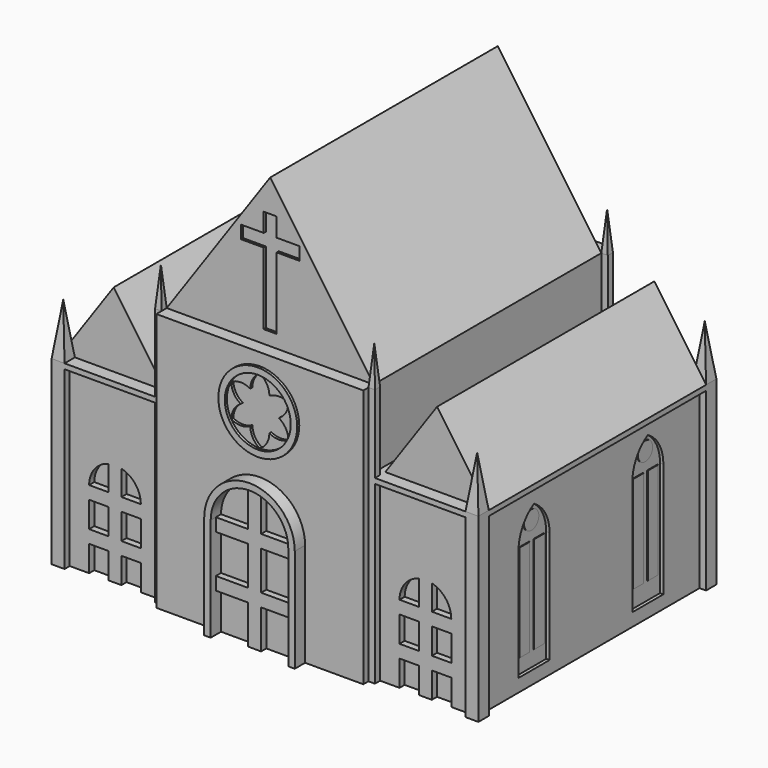
from build123d import *

# Parameters (mm, degrees)
F0_W      = 3.175
F0_H      = 3.175
F1_DEPTH  = 127
F2_DEPTH  = 88.9
F3_W      = 50.8
F3_H      = 146.05
F4_DEPTH  = 2.54
F5_W      = 3.175
F5_H      = 133.35
F5_W_2    = 44.45
F5_H_2    = 3.175
F6_DEPTH  = 2.54
F8_DEPTH  = 139.7
F10_DEPTH = 139.7
F12_DEPTH = 146.05
F13_DEPTH = 6.35
F14_DEPTH = 6.35
F15_DEPTH = 6.35
F17_DEPTH = 3.175
F19_DEPTH = 3.175
F21_DEPTH = 127
F23_DEPTH = 3.175
F25_DEPTH = 3.175
F27_DEPTH = 127
F29_DEPTH = 6.35
F31_DEPTH = 25.4
F33_DEPTH = 6.35
F35_DEPTH = 14.732
F37_DEPTH = 6.35
F39_DEPTH = 25.4
F41_DEPTH = 6.35
F43_DEPTH = 6.35
F45_DEPTH = 6.35
F47_DEPTH = 3.175
F48_W     = 6.35
F48_H     = 6.35
F48_H_2   = 9.202644515
F48_W_2   = 11.1125
F48_H_3   = 35.247355485
F49_DEPTH = 1.27
F50_R     = 19.3618203149
F51_DEPTH = 1.27
F53_DEPTH = 1.27
F54_W     = 9.525
F54_H     = 12.7
F55_DEPTH = 3.175
F56_W     = 9.525
F56_H     = 12.7
F57_DEPTH = 3.175
F58_W     = 6.35
F58_H     = 47.625
F58_R     = 4.5339
F60_DEPTH = 1.651
F59_W     = 6.35
F59_H     = 47.625
F59_R     = 4.5339
F61_DEPTH = 1.27
F62_DEPTH = 1.651
F63_DEPTH = 1.27
F64_W     = 6.35
F64_H     = 47.625
F64_R     = 4.5339
F66_DEPTH = 1.27
F67_DEPTH = 1.4224
F65_R     = 4.5339
F65_W     = 6.35
F65_H     = 47.625
F68_DEPTH = 1.27
F69_DEPTH = 1.4224
F71_DEPTH = 6.35
F70_W     = 19.05
F70_H     = 25.4
F72_DEPTH = 3.175


# Not quite as in the source:
# - a pattern or mirror of a feature is missing from the dataset's text; its kind, count and spacing are read off the source's solid


with BuildPart() as f1:
    # F0 (on Top) → F1 (new body)
    with BuildSketch(Plane.XY):
        Polygon((50.8, 76.2), (-50.8, 76.2), (-50.8, 73.025), (-50.8, 69.85), (-50.8, -69.85), (-50.8, -73.025), (-50.8, -76.2), (50.8, -76.2), (50.8, -73.025), (50.8, -69.85), (50.8, 69.85), (50.8, 73.025), align=None)
        with Locations((-52.3875, 71.4375)):
            Rectangle(F0_W, F0_H)
        with Locations((52.3875, 71.4375)):
            Rectangle(F0_W, F0_H)
        with Locations((-52.3875, -71.4375)):
            Rectangle(F0_W, F0_H)
        with Locations((52.3875, -71.4375)):
            Rectangle(F0_W, F0_H)
    extrude(amount=F1_DEPTH)

    # F0 (on Top) → F2 (join)
    with BuildSketch(Plane.XY):
        with Locations((-52.3875, -71.4375)):
            Rectangle(F0_W, F0_H)
        Polygon((50.8, 76.2), (-50.8, 76.2), (-50.8, 73.025), (-50.8, 69.85), (-50.8, -69.85), (-50.8, -73.025), (-50.8, -76.2), (50.8, -76.2), (50.8, -73.025), (50.8, -69.85), (50.8, 69.85), (50.8, 73.025), align=None)
        with Locations((-52.3875, 71.4375)):
            Rectangle(F0_W, F0_H)
        Polygon((53.975, 69.85), (50.8, 69.85), (50.8, -69.85), (53.975, -69.85), (98.425, -69.85), (98.425, -73.025), (104.775, -73.025), (104.775, -66.675), (101.6, -66.675), (101.6, 66.675), (104.775, 66.675), (104.775, 73.025), (98.425, 73.025), (98.425, 69.85), align=None)
        with Locations((52.3875, 71.4375)):
            Rectangle(F0_W, F0_H)
        Polygon((-50.8, -69.85), (-50.8, 69.85), (-53.975, 69.85), (-98.425, 69.85), (-98.425, 73.025), (-104.775, 73.025), (-104.775, 66.675), (-101.6, 66.675), (-101.6, -66.675), (-104.775, -66.675), (-104.775, -73.025), (-98.425, -73.025), (-98.425, -69.85), (-53.975, -69.85), align=None)
        with Locations((52.3875, -71.4375)):
            Rectangle(F0_W, F0_H)
    extrude(amount=F2_DEPTH)

    # F3 (on face) → F4 (join)
    with BuildSketch(Plane.XY.offset(88.9)):
        with Locations((-79.375, 0)):
            Rectangle(F3_W, F3_H)
    extrude(amount=-F4_DEPTH)

    # F5 (on face) → F6 (join)
    with BuildSketch(Plane.XY.offset(88.9)):
        Polygon((98.425, -73.025), (104.775, -73.025), (104.775, -66.675), (101.6, -66.675), (101.6, 66.675), (104.775, 66.675), (104.775, 73.025), (98.425, 73.025), (98.425, 69.85), (53.975, 69.85), (53.975, -69.85), (98.425, -69.85), align=None)
        with Locations((103.1875, 0)):
            Rectangle(F5_W, F5_H)
        with Locations((76.2, 71.4375)):
            Rectangle(F5_W_2, F5_H_2)
        with Locations((76.2, -71.4375)):
            Rectangle(F5_W_2, F5_H_2)
    extrude(amount=-F6_DEPTH)

    # F9 (on face) → F10 (join)
    with BuildSketch(Plane.XZ.offset(73.025)):
        Polygon((53.975, 88.9), (104.775, 88.9), (79.375, 125.3779728055), align=None)
    extrude(amount=-F10_DEPTH)

    # F11 (on face) → F12 (join)
    with BuildSketch(Plane.XZ.offset(76.2)):
        Polygon((0, 199.955945611), (-50.8, 127), (50.8, 127), align=None)
    extrude(amount=-F12_DEPTH)

    # F11 (on face) → F13 (cut)
    with BuildSketch(Plane.XZ.offset(76.2)):
        Polygon((0, 199.955945611), (-50.8, 127), (50.8, 127), align=None)
    extrude(amount=-F13_DEPTH, mode=Mode.SUBTRACT)

    # F9 (on face) → F15 (cut)
    with BuildSketch(Plane.XZ.offset(73.025)):
        Polygon((53.975, 88.9), (104.775, 88.9), (79.375, 125.3779728055), align=None)
    extrude(amount=-F15_DEPTH, mode=Mode.SUBTRACT)

    # F16 (on face) → F17 (join)
    with BuildSketch(Plane.XZ.offset(73.025)):
        Polygon((-52.3875, 145.9837389297), (-53.975, 127), (-50.8, 127), align=None)
    extrude(amount=-F17_DEPTH)

    # F18 (on face) → F19 (join)
    with BuildSketch(Plane.XZ.offset(73.025)):
        Polygon((52.3875, 145.9837389297), (50.8, 127), (53.975, 127), align=None)
    extrude(amount=-F19_DEPTH)

    # F20 (on face) → F21 (cut)
    with BuildSketch(Plane(origin=(-53.975, 0, 0), x_dir=(0, -1, 0), z_dir=(-1, 0, 0))):
        Polygon((69.85, 145.9837389297), (69.85, 127), (71.4375, 145.9837389297), align=None)
        Polygon((73.025, 145.9837389297), (71.4375, 145.9837389297), (73.025, 127), align=None)
    extrude(amount=-F21_DEPTH, mode=Mode.SUBTRACT)

    # F22 (on face) → F23 (join)
    with BuildSketch(Plane(origin=(0, 73.025, 0), x_dir=(-1, 0, 0), z_dir=(0, 1, 0))):
        Polygon((50.8, 127), (53.975, 127), (52.3875, 145.9837389297), align=None)
    extrude(amount=-F23_DEPTH)

    # F24 (on face) → F25 (join)
    with BuildSketch(Plane(origin=(0, 73.025, 0), x_dir=(-1, 0, 0), z_dir=(0, 1, 0))):
        Polygon((-52.3875, 145.9837389297), (-53.975, 127), (-50.8, 127), align=None)
    extrude(amount=-F25_DEPTH)

    # F26 (on face) → F27 (cut)
    with BuildSketch(Plane(origin=(-53.975, 0, 0), x_dir=(0, -1, 0), z_dir=(-1, 0, 0))):
        Polygon((-73.025, 127), (-71.4375, 145.9837389297), (-73.025, 145.9837389297), align=None)
        Polygon((-71.4375, 145.9837389297), (-69.85, 127), (-69.85, 145.9837389297), align=None)
    extrude(amount=-F27_DEPTH, mode=Mode.SUBTRACT)

    # F29_copies: F29 across plane


with BuildPart() as f8:
    # F7 (on face) → F8 (new body)
    with BuildSketch(Plane.XZ.offset(73.025)):
        Polygon((-79.375, 125.3779728055), (-104.775, 88.9), (-53.975, 88.9), align=None)
    extrude(amount=-F8_DEPTH)

    # F14 (cut): a face of the model
    f14_faces = [f8.faces().sort_by_distance(p)[0] for p in [
        (-79.375, -73.025, 101.0593242685),
    ]]
    extrude(f14_faces, amount=-F14_DEPTH, mode=Mode.SUBTRACT)


with BuildPart() as f29:
    # F28 (on face) → F29 (new body)
    with BuildSketch(Plane.XZ.offset(73.025)):
        Polygon((-101.6, 114.1007812379), (-104.775, 88.9), (-98.425, 88.9), align=None)
    extrude(amount=-F29_DEPTH)


with BuildPart() as f1_1:
    add(f1.part)
    add(f29.part.mirror(Plane(origin=(0, 0, 0), x_dir=(0, 0, 1), z_dir=(1, 0, 0))))

    # F36 (on face) → F37 (join)
    with BuildSketch(Plane.XZ.offset(73.025)):
        Polygon((98.425, 88.9), (104.775, 88.9), (101.6, 114.1007812379), align=None)
    extrude(amount=-F37_DEPTH)

    # F38 (on face) → F39 (cut)
    with BuildSketch(Plane.YZ.offset(104.775)):
        Polygon((-73.025, 114.1007812379), (-73.025, 88.9), (-69.85, 114.1007812379), align=None)
        Polygon((-66.675, 114.1007812379), (-69.85, 114.1007812379), (-66.675, 88.9), align=None)
    extrude(amount=-F39_DEPTH, mode=Mode.SUBTRACT)

    # F40 (on face) → F41 (join)
    with BuildSketch(Plane.YZ.offset(104.775)):
        Polygon((66.675, 88.9), (73.025, 88.9), (69.85, 114.1007812379), align=None)
    extrude(amount=-F41_DEPTH)

    # F42 (on face) → F43 (cut)
    with BuildSketch(Plane(origin=(0, 73.025, 0), x_dir=(-1, 0, 0), z_dir=(0, 1, 0))):
        Polygon((-104.775, 88.9), (-101.6, 114.1007812379), (-104.775, 114.1007812379), align=None)
        Polygon((-101.6, 114.1007812379), (-98.425, 88.9), (-98.425, 114.1007812379), align=None)
    extrude(amount=-F43_DEPTH, mode=Mode.SUBTRACT)

    # F44 (on face) → F45 (join)
    with BuildSketch(Plane.XZ.offset(76.2)):
        with BuildLine():
            Line((-22.225, 50.8), (-22.225, 0))
            Line((-22.225, 0), (-19.05, 0))
            Line((-19.05, 0), (-19.05, 50.8))
            ThreePointArc((-19.05, 50.8), (0, 69.85), (19.05, 50.8))
            Line((19.05, 50.8), (19.05, 0))
            Line((19.05, 0), (22.225, 0))
            Line((22.225, 0), (22.225, 50.8))
            ThreePointArc((22.225, 50.8), (0, 73.025), (-22.225, 50.8))
        make_face()
    extrude(amount=F45_DEPTH)

    # F46 (on face) → F47 (join)
    with BuildSketch(Plane.XZ.offset(76.2)):
        with BuildLine():
            Line((-3.175, 19.05), (-3.175, 0))
            Line((-3.175, 0), (3.175, 0))
            Line((3.175, 0), (3.175, 19.05))
            Line((3.175, 19.05), (19.05, 19.05))
            Line((19.05, 19.05), (19.05, 25.4))
            Line((19.05, 25.4), (3.175, 25.4))
            Line((3.175, 25.4), (3.175, 44.45))
            Line((3.175, 44.45), (19.05, 44.45))
            Line((19.05, 44.45), (19.05, 50.8))
            Line((19.05, 50.8), (3.175, 50.8))
            Line((3.175, 50.8), (3.175, 69.5835533113))
            ThreePointArc((3.175, 69.5835533113), (1.5930802583, 69.7832714591), (0, 69.85))
            ThreePointArc((0, 69.85), (-1.5930802583, 69.7832714591), (-3.175, 69.5835533113))
            Line((-3.175, 69.5835533113), (-3.175, 50.8))
            Line((-3.175, 50.8), (-19.05, 50.8))
            Line((-19.05, 50.8), (-19.05, 44.45))
            Line((-19.05, 44.45), (-3.175, 44.45))
            Line((-3.175, 44.45), (-3.175, 25.4))
            Line((-3.175, 25.4), (-19.05, 25.4))
            Line((-19.05, 25.4), (-19.05, 19.05))
            Line((-19.05, 19.05), (-3.175, 19.05))
        make_face()
    extrude(amount=F47_DEPTH)

    # F48 (on face) → F49 (cut)
    with BuildSketch(Plane.XZ.offset(69.85)):
        with Locations((0, 171.772355485)):
            Rectangle(F48_W, F48_H)
        with Locations((0, 179.5486777425)):
            Rectangle(F48_W, F48_H_2)
        with Locations((8.73125, 171.772355485)):
            Rectangle(F48_W_2, F48_H)
        with Locations((-8.73125, 171.772355485)):
            Rectangle(F48_W_2, F48_H)
        with Locations((0, 150.9736777425)):
            Rectangle(F48_W, F48_H_3)
    extrude(amount=-F49_DEPTH, mode=Mode.SUBTRACT)

    # F50 (on face) → F51 (join)
    with BuildSketch(Plane.XZ.offset(76.2)):
        with Locations((0, 101.6)):
            Circle(F50_R)
        with BuildLine():
            ThreePointArc((14.0181975992, 109.6934101575), (15.6352677877, 105.7894573772), (16.1868203149, 101.6))
            ThreePointArc((16.1868203149, 101.6), (15.6352677877, 97.4105426228), (14.0181975992, 93.5065898425))
            ThreePointArc((14.0181975992, 93.5065898425), (8.0934101575, 87.5818024008), (0, 85.4131796851))
            ThreePointArc((0, 85.4131796851), (-8.0934101575, 87.5818024008), (-14.0181975992, 93.5065898425))
            ThreePointArc((-14.0181975992, 93.5065898425), (-16.1868203149, 101.6), (-14.0181975992, 109.6934101575))
            ThreePointArc((-14.0181975992, 109.6934101575), (-8.0934101575, 115.6181975992), (0, 117.7868203149))
            ThreePointArc((0, 117.7868203149), (8.0934101575, 115.6181975992), (14.0181975992, 109.6934101575))
        make_face(mode=Mode.SUBTRACT)
    extrude(amount=F51_DEPTH)

    # F52 (on face) → F53 (cut)
    with BuildSketch(Plane.XZ.offset(76.2)):
        with BuildLine():
            ThreePointArc((-4.6727325331, 109.6934101575), (-9.3454650662, 110.9454650662), (-14.0181975992, 109.6934101575))
            ThreePointArc((-14.0181975992, 109.6934101575), (-12.7661426905, 105.0206776244), (-9.3454650662, 101.6))
            ThreePointArc((-9.3454650662, 101.6), (-4.6727325331, 102.8520549087), (0, 101.6))
            ThreePointArc((0, 101.6), (-3.4206776244, 105.0206776244), (-4.6727325331, 109.6934101575))
        make_face()
        with BuildLine():
            ThreePointArc((-4.6727325331, 109.6934101575), (-1.2520549087, 106.2727325331), (0, 101.6))
            ThreePointArc((0, 101.6), (1.2520549087, 106.2727325331), (4.6727325331, 109.6934101575))
            ThreePointArc((4.6727325331, 109.6934101575), (3.4206776244, 114.3661426905), (0, 117.7868203149))
            ThreePointArc((0, 117.7868203149), (-3.4206776244, 114.3661426905), (-4.6727325331, 109.6934101575))
        make_face()
        with BuildLine():
            ThreePointArc((-4.6727325331, 109.6934101575), (-3.4206776244, 105.0206776244), (0, 101.6))
            ThreePointArc((0, 101.6), (-1.2520549087, 106.2727325331), (-4.6727325331, 109.6934101575))
        make_face()
        with BuildLine():
            ThreePointArc((4.6727325331, 109.6934101575), (1.2520549087, 106.2727325331), (0, 101.6))
            ThreePointArc((0, 101.6), (3.4206776244, 105.0206776244), (4.6727325331, 109.6934101575))
        make_face()
        with BuildLine():
            ThreePointArc((9.3454650662, 101.6), (12.7661426905, 105.0206776244), (14.0181975992, 109.6934101575))
            ThreePointArc((14.0181975992, 109.6934101575), (9.3454650662, 110.9454650662), (4.6727325331, 109.6934101575))
            ThreePointArc((4.6727325331, 109.6934101575), (3.4206776244, 105.0206776244), (0, 101.6))
            ThreePointArc((0, 101.6), (4.6727325331, 102.8520549087), (9.3454650662, 101.6))
        make_face()
        with BuildLine():
            ThreePointArc((0, 101.6), (4.6727325331, 100.3479450913), (9.3454650662, 101.6))
            ThreePointArc((9.3454650662, 101.6), (4.6727325331, 102.8520549087), (0, 101.6))
        make_face()
        with BuildLine():
            ThreePointArc((4.6727325331, 93.5065898425), (9.3454650662, 92.2545349338), (14.0181975992, 93.5065898425))
            ThreePointArc((14.0181975992, 93.5065898425), (12.7661426905, 98.1793223756), (9.3454650662, 101.6))
            ThreePointArc((9.3454650662, 101.6), (4.6727325331, 100.3479450913), (0, 101.6))
            ThreePointArc((0, 101.6), (3.4206776244, 98.1793223756), (4.6727325331, 93.5065898425))
        make_face()
        with BuildLine():
            ThreePointArc((0, 101.6), (1.2520549087, 96.9272674669), (4.6727325331, 93.5065898425))
            ThreePointArc((4.6727325331, 93.5065898425), (3.4206776244, 98.1793223756), (0, 101.6))
        make_face()
        with BuildLine():
            ThreePointArc((-4.6727325331, 93.5065898425), (-3.4206776244, 88.8338573095), (0, 85.4131796851))
            ThreePointArc((0, 85.4131796851), (3.4206776244, 88.8338573095), (4.6727325331, 93.5065898425))
            ThreePointArc((4.6727325331, 93.5065898425), (1.2520549087, 96.9272674669), (0, 101.6))
            ThreePointArc((0, 101.6), (-1.2520549087, 96.9272674669), (-4.6727325331, 93.5065898425))
        make_face()
        with BuildLine():
            ThreePointArc((-9.3454650662, 101.6), (-12.7661426905, 98.1793223756), (-14.0181975992, 93.5065898425))
            ThreePointArc((-14.0181975992, 93.5065898425), (-9.3454650662, 92.2545349338), (-4.6727325331, 93.5065898425))
            ThreePointArc((-4.6727325331, 93.5065898425), (-3.4206776244, 98.1793223756), (0, 101.6))
            ThreePointArc((0, 101.6), (-4.6727325331, 100.3479450913), (-9.3454650662, 101.6))
        make_face()
        with BuildLine():
            ThreePointArc((0, 101.6), (-3.4206776244, 98.1793223756), (-4.6727325331, 93.5065898425))
            ThreePointArc((-4.6727325331, 93.5065898425), (-1.2520549087, 96.9272674669), (0, 101.6))
        make_face()
        with BuildLine():
            ThreePointArc((0, 101.6), (-4.6727325331, 102.8520549087), (-9.3454650662, 101.6))
            ThreePointArc((-9.3454650662, 101.6), (-4.6727325331, 100.3479450913), (0, 101.6))
        make_face()
    extrude(amount=-F53_DEPTH, mode=Mode.SUBTRACT)

    # F54 (on face) → F55 (cut)
    with BuildSketch(Plane.XZ.offset(69.85)):
        with BuildLine():
            ThreePointArc((73.025, 50.3967221242), (66.159768429, 45.8771299333), (63.5, 38.1))
            Line((63.5, 38.1), (73.025, 38.1))
            Line((73.025, 38.1), (73.025, 50.3967221242))
        make_face()
        with BuildLine():
            Line((79.375, 38.1), (88.9, 38.1))
            ThreePointArc((88.9, 38.1), (86.240231571, 45.8771299333), (79.375, 50.3967221242))
            Line((79.375, 50.3967221242), (79.375, 38.1))
        make_face()
        with Locations((68.2625, 25.4)):
            Rectangle(F54_W, F54_H)
        with Locations((84.1375, 25.4)):
            Rectangle(F54_W, F54_H)
        with Locations((68.2625, 6.35)):
            Rectangle(F54_W, F54_H)
        with Locations((84.1375, 6.35)):
            Rectangle(F54_W, F54_H)
    extrude(amount=-F55_DEPTH, mode=Mode.SUBTRACT)

    # F56 (on face) → F57 (cut)
    with BuildSketch(Plane.XZ.offset(69.85)):
        with BuildLine():
            ThreePointArc((-79.375, 50.3967221242), (-86.240231571, 45.8771299333), (-88.9, 38.1))
            Line((-88.9, 38.1), (-79.375, 38.1))
            Line((-79.375, 38.1), (-79.375, 50.3967221242))
        make_face()
        with BuildLine():
            Line((-73.025, 38.1), (-63.5, 38.1))
            ThreePointArc((-63.5, 38.1), (-66.159768429, 45.8771299333), (-73.025, 50.3967221242))
            Line((-73.025, 50.3967221242), (-73.025, 38.1))
        make_face()
        with Locations((-84.1375, 25.4)):
            Rectangle(F56_W, F56_H)
        with Locations((-68.2625, 25.4)):
            Rectangle(F56_W, F56_H)
        with Locations((-84.1375, 6.35)):
            Rectangle(F56_W, F56_H)
        with Locations((-68.2625, 6.35)):
            Rectangle(F56_W, F56_H)
    extrude(amount=-F57_DEPTH, mode=Mode.SUBTRACT)

    # F58 (on face) → F60 (cut)
    with BuildSketch(Plane.YZ.offset(101.6)):
        with BuildLine():
            Line((-44.45, 61.3211781338), (-44.45, 6.35))
            Line((-44.45, 6.35), (-25.4, 6.35))
            Line((-25.4, 6.35), (-25.4, 61.3211781338))
            ThreePointArc((-25.4, 61.3211781338), (-27.9522160579, 70.8461781338), (-34.925, 77.8189620759))
            ThreePointArc((-34.925, 77.8189620759), (-41.8977839421, 70.8461781338), (-44.45, 61.3211781338))
        make_face()
        with Locations((-39.1836256802, 37.5086781338)):
            Rectangle(F58_W, F58_H, mode=Mode.SUBTRACT)
        with Locations((-30.1298515022, 37.5086781338)):
            Rectangle(F58_W, F58_H, mode=Mode.SUBTRACT)
        with Locations((-34.925, 70.3889781338)):
            Circle(F58_R, mode=Mode.SUBTRACT)
    extrude(amount=-F60_DEPTH, mode=Mode.SUBTRACT)

    # F59 (on face) → F61 (cut)
    with BuildSketch(Plane.YZ.offset(101.6)):
        with Locations((30.6663743198, 38.801324065)):
            Rectangle(F59_W, F59_H)
        with Locations((34.925, 71.681624065)):
            Circle(F59_R)
        with Locations((39.7201484978, 38.801324065)):
            Rectangle(F59_W, F59_H)
    extrude(amount=-F61_DEPTH, mode=Mode.SUBTRACT)

    # F59 (on face) → F62 (cut)
    with BuildSketch(Plane.YZ.offset(101.6)):
        with BuildLine():
            Line((25.4, 62.613824065), (25.4, 6.35))
            Line((25.4, 6.35), (44.45, 6.35))
            Line((44.45, 6.35), (44.45, 62.613824065))
            ThreePointArc((44.45, 62.613824065), (41.8977839421, 72.138824065), (34.925, 79.1116080071))
            ThreePointArc((34.925, 79.1116080071), (27.9522160579, 72.138824065), (25.4, 62.613824065))
        make_face()
        with Locations((30.6663743198, 38.801324065)):
            Rectangle(F59_W, F59_H, mode=Mode.SUBTRACT)
        with Locations((39.7201484978, 38.801324065)):
            Rectangle(F59_W, F59_H, mode=Mode.SUBTRACT)
        with Locations((34.925, 71.681624065)):
            Circle(F59_R, mode=Mode.SUBTRACT)
    extrude(amount=-F62_DEPTH, mode=Mode.SUBTRACT)

    # F58 (on face) → F63 (cut)
    with BuildSketch(Plane.YZ.offset(101.6)):
        with Locations((-30.1298515022, 37.5086781338)):
            Rectangle(F58_W, F58_H)
        with Locations((-39.1836256802, 37.5086781338)):
            Rectangle(F58_W, F58_H)
        with Locations((-34.925, 70.3889781338)):
            Circle(F58_R)
    extrude(amount=-F63_DEPTH, mode=Mode.SUBTRACT)

    # F64 (on face) → F66 (cut)
    with BuildSketch(Plane(origin=(-101.6, 0, 0), x_dir=(0, -1, 0), z_dir=(-1, 0, 0))):
        with Locations((30.6663743198, 36.1047450602)):
            Rectangle(F64_W, F64_H)
        with Locations((39.7201484978, 36.1047450602)):
            Rectangle(F64_W, F64_H)
        with Locations((34.925, 68.9850450602)):
            Circle(F64_R)
    extrude(amount=-F66_DEPTH, mode=Mode.SUBTRACT)

    # F64 (on face) → F67 (cut)
    with BuildSketch(Plane(origin=(-101.6, 0, 0), x_dir=(0, -1, 0), z_dir=(-1, 0, 0))):
        with BuildLine():
            Line((25.4, 59.9172450602), (25.4, 6.35))
            Line((25.4, 6.35), (44.45, 6.35))
            Line((44.45, 6.35), (44.45, 59.9172450602))
            ThreePointArc((44.45, 59.9172450602), (41.8977839421, 69.4422450602), (34.925, 76.4150290023))
            ThreePointArc((34.925, 76.4150290023), (27.9522160579, 69.4422450602), (25.4, 59.9172450602))
        make_face()
        with Locations((30.6663743198, 36.1047450602)):
            Rectangle(F64_W, F64_H, mode=Mode.SUBTRACT)
        with Locations((39.7201484978, 36.1047450602)):
            Rectangle(F64_W, F64_H, mode=Mode.SUBTRACT)
        with Locations((34.925, 68.9850450602)):
            Circle(F64_R, mode=Mode.SUBTRACT)
    extrude(amount=-F67_DEPTH, mode=Mode.SUBTRACT)

    # F65 (on face) → F68 (cut)
    with BuildSketch(Plane(origin=(-101.6, 0, 0), x_dir=(0, -1, 0), z_dir=(-1, 0, 0))):
        with Locations((-34.925, 70.0212035057)):
            Circle(F65_R)
        with Locations((-39.1836256802, 37.1409035057)):
            Rectangle(F65_W, F65_H)
        with Locations((-30.1298515022, 37.1409035057)):
            Rectangle(F65_W, F65_H)
    extrude(amount=-F68_DEPTH, mode=Mode.SUBTRACT)

    # F65 (on face) → F69 (cut)
    with BuildSketch(Plane(origin=(-101.6, 0, 0), x_dir=(0, -1, 0), z_dir=(-1, 0, 0))):
        with BuildLine():
            Line((-44.45, 60.9534035057), (-44.45, 6.35))
            Line((-44.45, 6.35), (-25.4, 6.35))
            Line((-25.4, 6.35), (-25.4, 60.9534035057))
            ThreePointArc((-25.4, 60.9534035057), (-27.9522160579, 70.4784035057), (-34.925, 77.4511874478))
            ThreePointArc((-34.925, 77.4511874478), (-41.8977839421, 70.4784035057), (-44.45, 60.9534035057))
        make_face()
        with Locations((-39.1836256802, 37.1409035057)):
            Rectangle(F65_W, F65_H, mode=Mode.SUBTRACT)
        with Locations((-30.1298515022, 37.1409035057)):
            Rectangle(F65_W, F65_H, mode=Mode.SUBTRACT)
        with Locations((-34.925, 70.0212035057)):
            Circle(F65_R, mode=Mode.SUBTRACT)
    extrude(amount=-F69_DEPTH, mode=Mode.SUBTRACT)

    # F70 (on face) → F71 (join)
    with BuildSketch(Plane(origin=(0, 76.2, 0), x_dir=(-1, 0, 0), z_dir=(0, 1, 0))):
        with BuildLine():
            Line((50.8, 69.85), (50.8, 76.2))
            ThreePointArc((50.8, 76.2), (35.921024463, 112.1210245055), (-6.01e-08, 127))
            ThreePointArc((-6.01e-08, 127), (-35.9210245055, 112.121024463), (-50.8, 76.2))
            Line((-50.8, 76.2), (-50.8, 69.85))
            Line((-50.8, 69.85), (50.8, 69.85))
        make_face()
        with BuildLine():
            Line((0, 76.2), (-47.625, 76.2))
            ThreePointArc((-47.625, 76.2), (-46.8245228219, 84.8950956004), (-44.45, 93.2978982627))
            ThreePointArc((-44.45, 93.2978982627), (-41.6720120833, 99.2561062178), (-38.1, 104.775))
            ThreePointArc((-38.1, 104.775), (-36.8330160341, 106.3905540663), (-35.4975791428, 107.95))
            ThreePointArc((-35.4975791428, 107.95), (-30.7464730948, 112.5702490675), (-25.4, 116.4862336909))
            ThreePointArc((-25.4, 116.4862336909), (-23.8301672635, 117.4342546094), (-22.225, 118.3211348375))
            ThreePointArc((-22.225, 118.3211348375), (-12.9836192496, 122.0210241721), (-3.175, 123.719048812))
            ThreePointArc((-3.175, 123.719048812), (0, 123.825), (3.175, 123.719048812))
            ThreePointArc((3.175, 123.719048812), (12.9836192496, 122.0210241721), (22.225, 118.3211348375))
            ThreePointArc((22.225, 118.3211348375), (23.8301672635, 117.4342546094), (25.4, 116.4862336909))
            ThreePointArc((25.4, 116.4862336909), (30.7464730948, 112.5702490675), (35.4975791428, 107.95))
            ThreePointArc((35.4975791428, 107.95), (36.8330160341, 106.3905540663), (38.1, 104.775))
            ThreePointArc((38.1, 104.775), (41.6720120833, 99.2561062178), (44.45, 93.2978982627))
            ThreePointArc((44.45, 93.2978982627), (46.8245228219, 84.8950956004), (47.625, 76.2))
            Line((47.625, 76.2), (0, 76.2))
        make_face(mode=Mode.SUBTRACT)
    extrude(amount=F71_DEPTH)

    # F70 (on face) → F72 (cut)
    with BuildSketch(Plane(origin=(0, 76.2, 0), x_dir=(-1, 0, 0), z_dir=(0, 1, 0))):
        with Locations((12.7, 92.075)):
            Rectangle(F70_W, F70_H)
        with BuildLine():
            Line((22.225, 107.95), (22.225, 118.3211348375))
            ThreePointArc((22.225, 118.3211348375), (12.9836192496, 122.0210241721), (3.175, 123.719048812))
            Line((3.175, 123.719048812), (3.175, 107.95))
            Line((3.175, 107.95), (22.225, 107.95))
        make_face()
        with BuildLine():
            ThreePointArc((-3.175, 123.719048812), (-12.9836192496, 122.0210241721), (-22.225, 118.3211348375))
            Line((-22.225, 118.3211348375), (-22.225, 107.95))
            Line((-22.225, 107.95), (-3.175, 107.95))
            Line((-3.175, 107.95), (-3.175, 123.719048812))
        make_face()
        with BuildLine():
            ThreePointArc((-25.4, 116.4862336909), (-30.7464730948, 112.5702490675), (-35.4975791428, 107.95))
            Line((-35.4975791428, 107.95), (-25.4, 107.95))
            Line((-25.4, 107.95), (-25.4, 116.4862336909))
        make_face()
        with BuildLine():
            ThreePointArc((-38.1, 104.775), (-41.6720120833, 99.2561062178), (-44.45, 93.2978982627))
            Line((-44.45, 93.2978982627), (-44.45, 79.375))
            Line((-44.45, 79.375), (-25.4, 79.375))
            Line((-25.4, 79.375), (-25.4, 104.775))
            Line((-25.4, 104.775), (-38.1, 104.775))
        make_face()
        with Locations((-12.7, 92.075)):
            Rectangle(F70_W, F70_H)
        with BuildLine():
            Line((25.4, 107.95), (35.4975791428, 107.95))
            ThreePointArc((35.4975791428, 107.95), (30.7464730948, 112.5702490675), (25.4, 116.4862336909))
            Line((25.4, 116.4862336909), (25.4, 107.95))
        make_face()
        with BuildLine():
            Line((44.45, 79.375), (44.45, 93.2978982627))
            ThreePointArc((44.45, 93.2978982627), (41.6720120833, 99.2561062178), (38.1, 104.775))
            Line((38.1, 104.775), (25.4, 104.775))
            Line((25.4, 104.775), (25.4, 79.375))
            Line((25.4, 79.375), (44.45, 79.375))
        make_face()
    extrude(amount=-F72_DEPTH, mode=Mode.SUBTRACT)


with BuildPart() as f29_1:
    add(f29.part)

    # F30 (on face) → F31 (cut)
    with BuildSketch(Plane(origin=(-104.775, 0, 0), x_dir=(0, -1, 0), z_dir=(-1, 0, 0))):
        Polygon((73.025, 114.1007812379), (69.85, 114.1007812379), (73.025, 88.9), align=None)
        Polygon((66.675, 114.1007812379), (66.675, 88.9), (69.85, 114.1007812379), align=None)
    extrude(amount=-F31_DEPTH, mode=Mode.SUBTRACT)


with BuildPart() as f33:
    # F32 (on face) → F33 (new body)
    with BuildSketch(Plane(origin=(0, 73.025, 0), x_dir=(-1, 0, 0), z_dir=(0, 1, 0))):
        Polygon((98.425, 88.9), (104.775, 88.9), (101.6, 114.1007812379), align=None)
    extrude(amount=-F33_DEPTH)

    # F34 (on face) → F35 (cut)
    with BuildSketch(Plane(origin=(-104.775, 0, 0), x_dir=(0, -1, 0), z_dir=(-1, 0, 0))):
        Polygon((-73.025, 88.9), (-69.85, 114.1007812379), (-73.025, 114.1007812379), align=None)
        Polygon((-69.85, 114.1007812379), (-66.675, 88.9), (-66.675, 114.1007812379), align=None)
    extrude(amount=-F35_DEPTH, mode=Mode.SUBTRACT)


solid = Compound([f8.part, f1_1.part, f29_1.part, f33.part])
